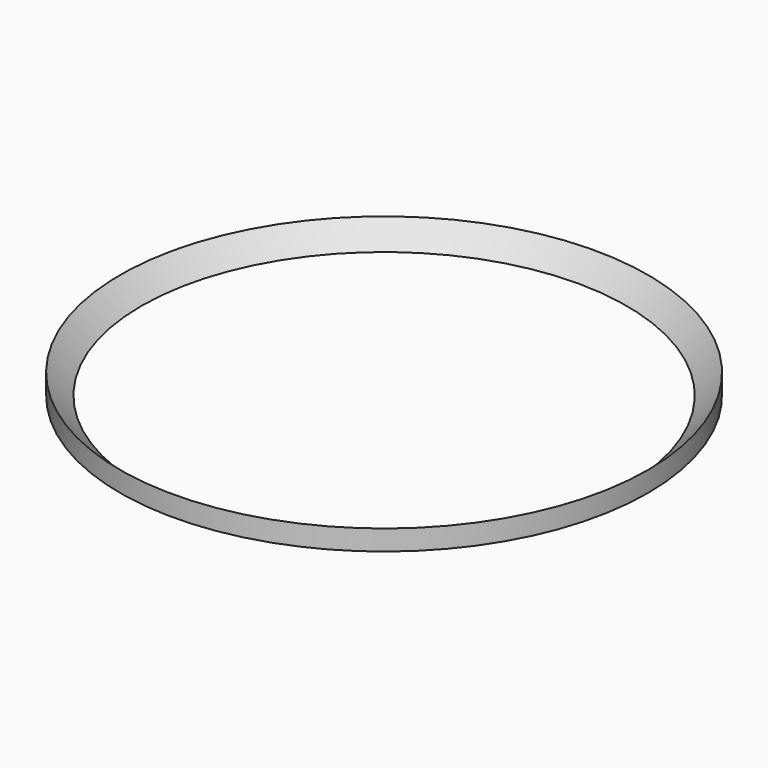
from build123d import *


# Not quite as in the source:
# - the program builds the solid bodies; features that only make, move or delete a surface that nothing else refers to are left out


with BuildPart() as f4:
    # F2 (on Front) → F4 (revolve)
    with BuildSketch(Plane.XZ):
        Polygon((202.22, 0), (220, 0), (220, 16.9331612126), align=None)
    revolve(axis=Axis((0, 0, 31.6398665309), (0, 0, 1)))


solid = f4.part
